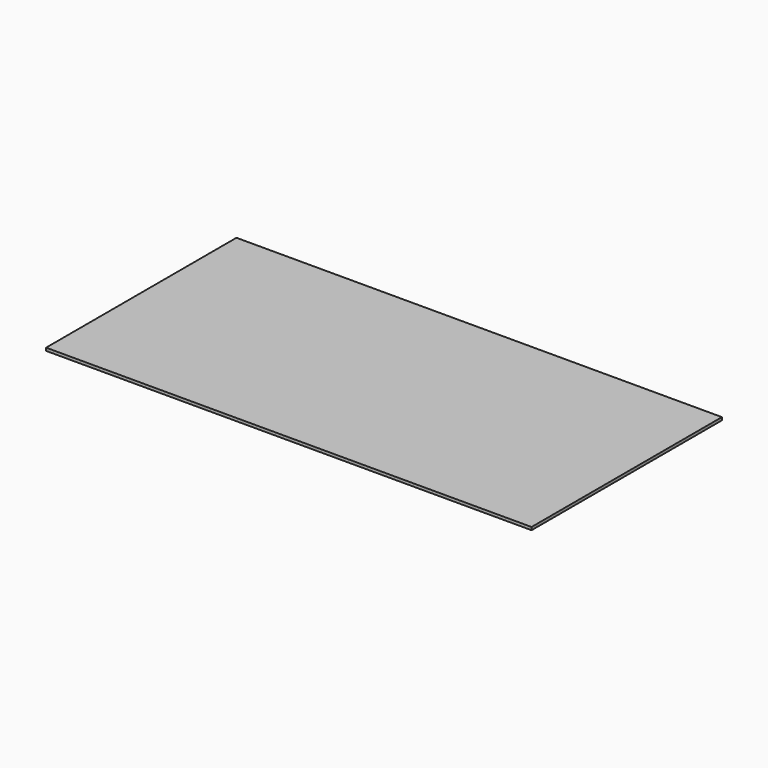
from build123d import *

# Parameters (mm, degrees)
F0_W     = 805.815
F0_H     = 394.97
F1_DEPTH = 4.7625


# Not quite as in the source:
# - a length typed as a fraction of an inch, garbled in the dataset ("3 / 203.2 mm" for 3/8 in), is restored


with BuildPart() as f1:
    # F0 (on Top) → F1 (new body)
    with BuildSketch(Plane.XY):
        Rectangle(F0_W, F0_H)
    extrude(amount=F1_DEPTH)


solid = f1.part
